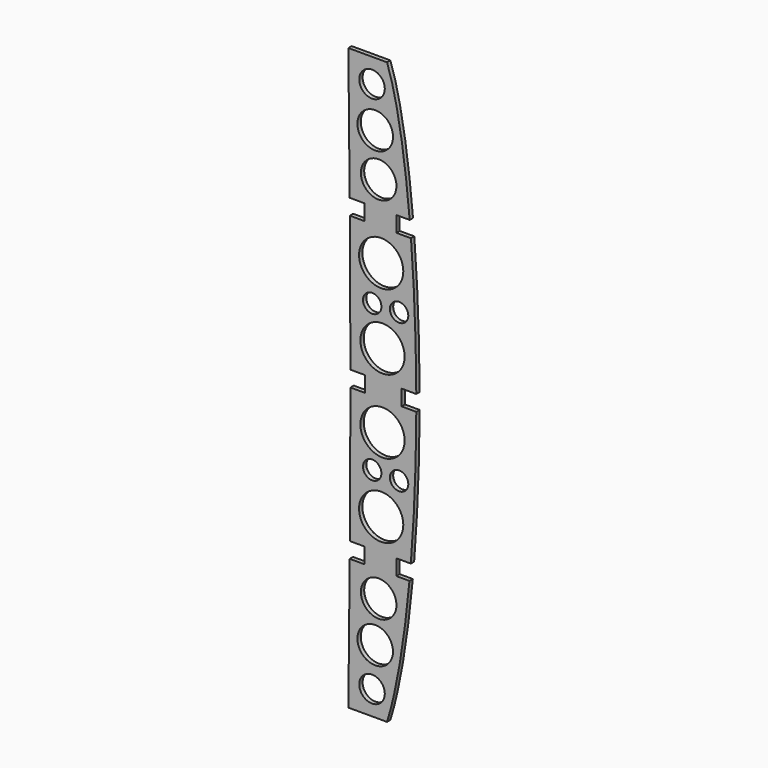
from build123d import *

# Parameters (mm, degrees)
F0_R     = 21.1586469213
F0_R_2   = 8.806010366
F0_R_3   = 12.2091210128
F0_R_4   = 17.006361888
F1_DEPTH = 4


# Not quite as in the source:
# - ends of sketch curves that miss each other by under 0.0002 mm in the source are joined


with BuildPart() as f1:
    # F0 (on Front) → F1 (new body)
    with BuildSketch(Plane.XZ):
        with BuildLine():
            Line((-404.2813370244, -555.8222100041), (-369.2932587578, -555.8222100041))
            Line((-369.2932587578, -555.8222100041), (-369.2932587578, -548.3222100041))
            Line((-369.2932587578, -548.3222100041), (-355.2932587578, -548.3222100041))
            add(Edge.make_bspline(
                [(-360.3678395822, -418.8222100041), (-357.2043853814, -459.4781491099), (-355.4697568796, -504.0564149856), (-355.2932587578, -548.3222100041)],
                knots=[0.2913303101, 0.2913303101, 0.2913303101, 0.2913303101, 0.4888396728, 0.4888396728, 0.4888396728, 0.4888396728], degree=3))
            Line((-360.3678395822, -418.8222100041), (-374.3678395822, -418.8222100041))
            Line((-374.3678395822, -418.8222100041), (-374.3678395822, -411.3222100041))
            Line((-374.3678395822, -411.3222100041), (-404.8922608862, -411.3222100041))
            Line((-404.8922608862, -411.3222100041), (-404.8922608862, -418.8222100041))
            Line((-404.8922608862, -418.8222100041), (-418.8922608862, -418.8222100041))
            add(Edge.make_bspline(
                [(-418.8922608862, -418.8222100041), (-418.5472091576, -461.9778150808), (-418.3109664436, -505.1392537968), (-418.2813370244, -548.3222100041)],
                knots=[0.2533782445, 0.2533782445, 0.2533782445, 0.2533782445, 0.4865039964, 0.4865039964, 0.4865039964, 0.4865039964], degree=3))
            Line((-418.2813370244, -548.3222100041), (-404.2813370244, -548.3222100041))
            Line((-404.2813370244, -548.3222100041), (-404.2813370244, -555.8222100041))
        make_face()
        with Locations((-387.5988423824, -520.4372406006)):
            Circle(F0_R, mode=Mode.SUBTRACT)
        with Locations((-397.4644243717, -485.6480360031)):
            Circle(F0_R_2, mode=Mode.SUBTRACT)
        with Locations((-371.7619478703, -484.8691523075)):
            Circle(F0_R_2, mode=Mode.SUBTRACT)
        with Locations((-388.8969421387, -449.0414857864)):
            Circle(F0_R, mode=Mode.SUBTRACT)
        with BuildLine():
            Line((-369.2932587578, -563.3222100041), (-369.2932587578, -555.8222100041))
            Line((-369.2932587578, -555.8222100041), (-404.2813370244, -555.8222100041))
            Line((-404.2813370244, -555.8222100041), (-404.2813370244, -563.3222100041))
            Line((-404.2813370244, -563.3222100041), (-418.2794696915, -563.3222100041))
            add(Edge.make_bspline(
                [(-418.2794696915, -563.3222100041), (-418.2983515169, -606.4848543261), (-418.524010714, -649.6671773036), (-418.8658189061, -692.8222100041)],
                knots=[0.5134952141, 0.5134952141, 0.5134952141, 0.5134952141, 0.746484428, 0.746484428, 0.746484428, 0.746484428], degree=3))
            Line((-418.8658189061, -692.8222100041), (-404.8922608862, -692.8222100041))
            Line((-404.8922608862, -692.8222100041), (-404.8922608862, -700.3222100041))
            Line((-404.8922608862, -700.3222100041), (-374.3678395822, -700.3222100041))
            Line((-374.3678395822, -700.3222100041), (-374.3678395822, -692.8222100041))
            Line((-374.3678395822, -692.8222100041), (-360.5407278397, -692.8222100041))
            add(Edge.make_bspline(
                [(-355.2933001029, -563.3222098386), (-355.473221284, -608.2616104093), (-357.267833957, -652.4575821746), (-360.5407278397, -692.8222100041)],
                knots=[0.5111757389, 0.5111757389, 0.5111757389, 0.5111757389, 0.7122386539, 0.7122386539, 0.7122386539, 0.7122386539], degree=3))
            Line((-355.2933001029, -563.3222098386), (-369.2932587578, -563.3222100041))
        make_face()
        with Locations((-388.8969421387, -662.6029342218)):
            Circle(F0_R, mode=Mode.SUBTRACT)
        with Locations((-397.4644243717, -625.9963840052)):
            Circle(F0_R_2, mode=Mode.SUBTRACT)
        with Locations((-371.7619478703, -626.7752677008)):
            Circle(F0_R_2, mode=Mode.SUBTRACT)
        with Locations((-387.5988423824, -591.2071794077)):
            Circle(F0_R, mode=Mode.SUBTRACT)
        with BuildLine():
            add(Edge.make_bspline(
                [(-361.8416139057, -707.8222100042), (-366.5966911813, -759.211500512), (-373.8431834552, -803.4077276906), (-383.2773775989, -833.5357473143)],
                knots=[0.7374547732, 0.7374547732, 0.7374547732, 0.7374547732, 1, 1, 1, 1], degree=3))
            Line((-361.8416139057, -707.8222100041), (-374.3678395822, -707.8222100041))
            Line((-374.3678395822, -707.8222100041), (-374.3678395822, -700.3222100041))
            Line((-374.3678395822, -700.3222100041), (-404.8922608862, -700.3222100041))
            Line((-404.8922608862, -700.3222100041), (-404.8922608862, -707.8222100041))
            Line((-404.8922608862, -707.8222100041), (-418.8922608862, -707.8222100041))
            Line((-418.8922608862, -707.8222100041), (-418.9891725019, -707.8222100041))
            add(Edge.make_bspline(
                [(-418.9891725019, -707.8222100041), (-419.3464745558, -749.7720501318), (-419.8036381759, -791.690950422), (-420.2773775989, -833.5357473143)],
                knots=[0.7734809807, 0.7734809807, 0.7734809807, 0.7734809807, 1, 1, 1, 1], degree=3))
            Line((-420.2773775989, -833.5357473143), (-383.2773775989, -833.5357473143))
        make_face()
        with Locations((-397.6303637028, -810.5115026041)):
            Circle(F0_R_3, mode=Mode.SUBTRACT)
        with Locations((-394.5856392384, -772.5696891352)):
            Circle(F0_R_4, mode=Mode.SUBTRACT)
        with Locations((-391.3067281246, -732.2857707544)):
            Circle(F0_R_4, mode=Mode.SUBTRACT)
        with BuildLine():
            Line((-404.8922608862, -411.3222100041), (-374.3678395822, -411.3222100041))
            Line((-374.3678395822, -411.3222100041), (-374.3678395822, -403.8222100041))
            Line((-374.3678395822, -403.8222100041), (-361.6160762359, -403.8222100041))
            add(Edge.make_bspline(
                [(-383.2773775989, -278.108672694), (-373.6927686449, -304.944377163), (-366.3661772603, -350.3256078146), (-361.6160762359, -403.8222100042)],
                knots=[0, 0, 0, 0, 0.2667311371, 0.2667311371, 0.2667311371, 0.2667311371], degree=3))
            Line((-383.2773775989, -278.108672694), (-420.2773775989, -278.108672694))
            add(Edge.make_bspline(
                [(-420.2773775989, -278.108672694), (-419.8248476428, -320.0189708532), (-419.3746825014, -361.9186969271), (-419.0164252465, -403.8222100041)],
                knots=[0, 0, 0, 0, 0.2263679612, 0.2263679612, 0.2263679612, 0.2263679612], degree=3))
            Line((-419.0164252465, -403.8222100041), (-418.8922608862, -403.8222100041))
            Line((-418.8922608862, -403.8222100041), (-404.8922608862, -403.8222100041))
            Line((-404.8922608862, -403.8222100041), (-404.8922608862, -411.3222100041))
        make_face()
        with Locations((-391.3067281246, -379.3586492538)):
            Circle(F0_R_4, mode=Mode.SUBTRACT)
        with Locations((-394.5856392384, -339.0747308731)):
            Circle(F0_R_4, mode=Mode.SUBTRACT)
        with Locations((-397.6303637028, -301.1329174042)):
            Circle(F0_R_3, mode=Mode.SUBTRACT)
    extrude(amount=F1_DEPTH)


solid = f1.part
